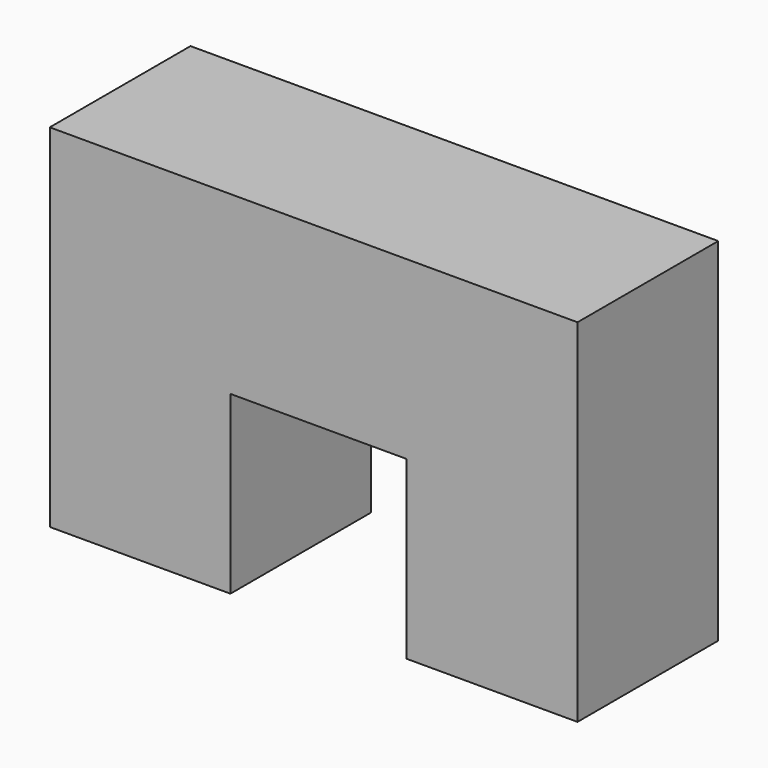
from build123d import *

# Parameters (mm, degrees)
F1_W     = 228.6
F1_H     = 152.4
F2_DEPTH = 76.2
F3_W     = 76.2
F3_H     = 76.2
F4_DEPTH = 76.201


# Not quite as in the source:
# - a variable given as a bare number and used for a length is read in inches; the dataset says mm whatever the document's units were


with BuildPart() as f2:
    # F1 (on Front) → F2 (new body)
    with BuildSketch(Plane.XZ):
        Rectangle(F1_W, F1_H)
    extrude(amount=F2_DEPTH)

    # F3 (on face) → F4 (cut, through all)
    with BuildSketch(Plane.XZ.offset(76.2)):
        with Locations((2.0580249786, -38.1)):
            Rectangle(F3_W, F3_H)
    extrude(amount=-F4_DEPTH, mode=Mode.SUBTRACT)


solid = f2.part
